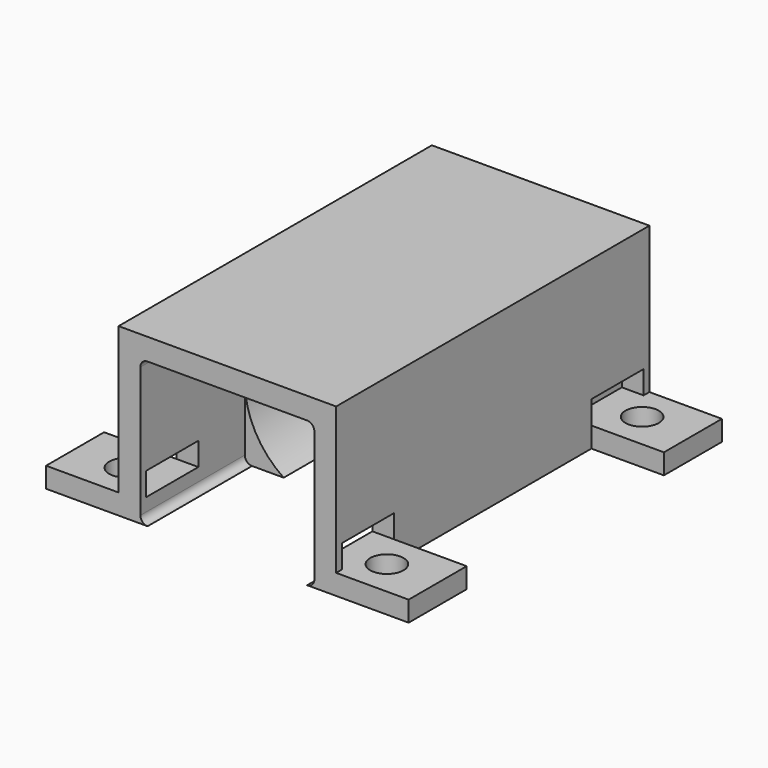
from build123d import *

# Parameters (mm, degrees)
F0_W      = 15
F0_H      = 11.5
F1_DEPTH  = 27
F3_DEPTH  = 9
F5_DEPTH  = 15
F7_DEPTH  = 3
F8_W      = 5
F8_H      = 1.4
F9_DEPTH  = 5
F10_R     = 1.15
F11_DEPTH = 1.4
F12_W     = 4.5
F12_H     = 1.6
F13_DEPTH = 1.5
F14_W     = 5
F14_H     = 1.4
F15_DEPTH = 5
F16_R     = 1.15
F17_DEPTH = 1.4
F18_W     = 4.5
F18_H     = 1.6
F19_DEPTH = 1.5


# Not quite as in the source:
# - a feature names something its author has since deleted; it is built from what else it names


with BuildPart() as f1:
    # F0 (on Front) → F1 (new body)
    with BuildSketch(Plane.XZ):
        with Locations((0, 0.75)):
            Rectangle(F0_W, F0_H)
    extrude(amount=-F1_DEPTH)

    # F2 (on Front) → F3 (cut)
    with BuildSketch(Plane.XZ):
        with BuildLine():
            Line((5.5, 5), (-5.5, 5))
            ThreePointArc((-5.5, 5), (-5.8535533906, 4.8535533906), (-6, 4.5))
            Line((-6, 4.5), (-6, -4.5))
            ThreePointArc((-6, -4.5), (-5.8535533906, -4.8535533906), (-5.5, -5))
            Line((-5.5, -5), (5.5, -5))
            ThreePointArc((5.5, -5), (5.8535533906, -4.8535533906), (6, -4.5))
            Line((6, -4.5), (6, 4.5))
            ThreePointArc((6, 4.5), (5.8535533906, 4.8535533906), (5.5, 5))
        make_face()
    extrude(amount=-F3_DEPTH, mode=Mode.SUBTRACT)

    # F4 (on face) → F5 (cut)
    with BuildSketch(Plane.XZ.offset(-9)):
        with BuildLine():
            Line((-3.3166247904, -5), (3.3166247904, -5))
            ThreePointArc((3.3166247904, -5), (5.2867640737, -2.8372743309), (6, 0))
            ThreePointArc((6, 0), (5.2867640737, 2.8372743309), (3.3166247904, 5))
            Line((3.3166247904, 5), (0, 5))
            Line((0, 5), (-3.3166247904, 5))
            ThreePointArc((-3.3166247904, 5), (-5.2867640737, 2.8372743309), (-6, 0))
            ThreePointArc((-6, 0), (-5.2867640737, -2.8372743309), (-3.3166247904, -5))
        make_face()
    extrude(amount=-F5_DEPTH, mode=Mode.SUBTRACT)

    # F6 (on face) → F7 (cut)
    with BuildSketch(Plane.XZ.offset(-24)):
        with BuildLine():
            ThreePointArc((4.8733971724, -3.5), (5.7114088907, -1.8384255445), (6, 0))
            ThreePointArc((6, 0), (5.7114088907, 1.8384255445), (4.8733971724, 3.5))
            Line((4.8733971724, 3.5), (0, 3.5))
            Line((0, 3.5), (-4.8733971724, 3.5))
            ThreePointArc((-4.8733971724, 3.5), (-6, 0), (-4.8733971724, -3.5))
            Line((-4.8733971724, -3.5), (4.8733971724, -3.5))
        make_face()
    extrude(amount=-F7_DEPTH, mode=Mode.SUBTRACT)

    # F8 (on face) → F9 (join)
    with BuildSketch(Plane.YZ.offset(7.5)):
        with Locations((2.5, -4.3)):
            Rectangle(F8_W, F8_H)
        with Locations((24.5, -4.3)):
            Rectangle(F8_W, F8_H)
    extrude(amount=F9_DEPTH)

    # F10 (on face) → F11 (cut)
    with BuildSketch(Plane.XY.offset(-3.6)):
        with Locations((9, 24.5)):
            Circle(F10_R)
        with Locations((9, 2.5)):
            Circle(F10_R)
    extrude(amount=-F11_DEPTH, mode=Mode.SUBTRACT)

    # F12 (on face) → F13 (cut)
    with BuildSketch(Plane.YZ.offset(7.5)):
        with Locations((2.75, -2.8)):
            Rectangle(F12_W, F12_H)
        with Locations((24.25, -2.8)):
            Rectangle(F12_W, F12_H)
    extrude(amount=-F13_DEPTH, mode=Mode.SUBTRACT)

    # F14 (on face) → F15 (join)
    with BuildSketch(Plane(origin=(-7.5, 0, 0), x_dir=(0, -1, 0), z_dir=(-1, 0, 0))):
        with Locations((-24.5, -4.3)):
            Rectangle(F14_W, F14_H)
        with Locations((-2.5, -4.3)):
            Rectangle(F14_W, F14_H)
    extrude(amount=F15_DEPTH)

    # F16 (on face) → F17 (cut)
    with BuildSketch(Plane.XY.offset(-3.6)):
        with Locations((-9, 2.5)):
            Circle(F16_R)
        with Locations((-9, 24.5)):
            Circle(F16_R)
    extrude(amount=-F17_DEPTH, mode=Mode.SUBTRACT)

    # F18 (on face) → F19 (cut)
    with BuildSketch(Plane(origin=(-7.5, 0, 0), x_dir=(0, -1, 0), z_dir=(-1, 0, 0))):
        with Locations((-24.25, -2.8)):
            Rectangle(F18_W, F18_H)
        with Locations((-2.75, -2.8)):
            Rectangle(F18_W, F18_H)
    extrude(amount=-F19_DEPTH, mode=Mode.SUBTRACT)


solid = f1.part
